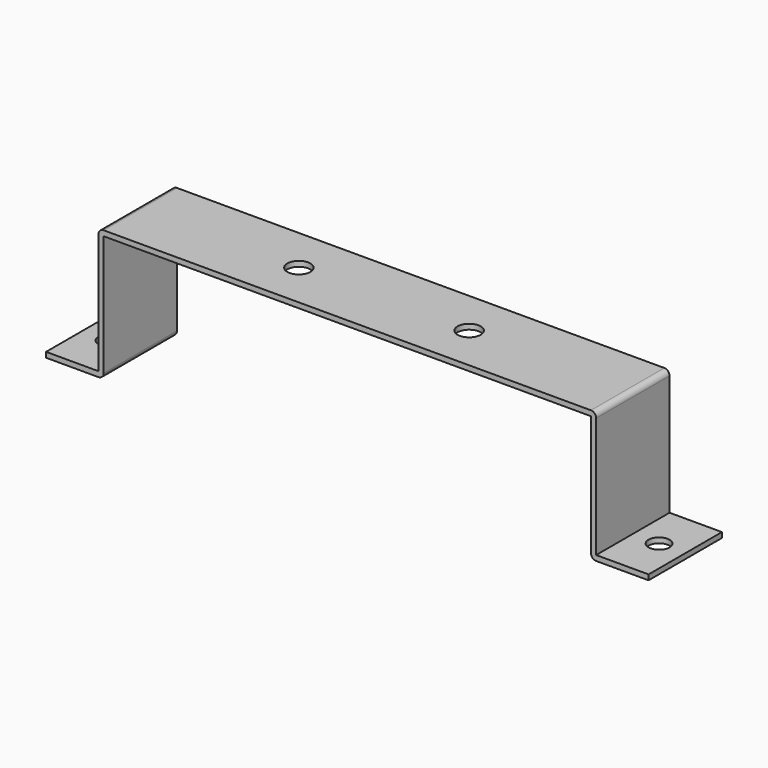
from build123d import *

# Parameters (mm, degrees)
F1_DEPTH = 17.5
F2_R     = 4
F3_DEPTH = 25
F4_R     = 4.4
F5_DEPTH = 25
F6_R     = 2


# Not quite as in the source:
# - a feature names something its author has since deleted; it is built from what else it names


with BuildPart() as f1:
    # F0 (on Front) → F1 (new body, symmetric)
    with BuildSketch(Plane.XZ):
        Polygon((95, -38), (95, 10), (-95, 10), (-95, -38), (-115, -38), (-115, -40), (-93, -40), (-93, 8), (93, 8), (93, -40), (115, -40), (115, -38), align=None)
    extrude(amount=F1_DEPTH, both=True)

    # F2 (on face) → F3 (cut)
    with BuildSketch(Plane.XY.offset(-38)):
        with Locations((-105, 0)):
            Circle(F2_R)
        with Locations((105, 0)):
            Circle(F2_R)
    extrude(amount=-F3_DEPTH, mode=Mode.SUBTRACT)

    # F4 (on face) → F5 (cut)
    with BuildSketch(Plane.XY.offset(10)):
        with Locations((-32.5, 0)):
            Circle(F4_R)
        with Locations((32.5, 0)):
            Circle(F4_R)
    extrude(amount=-F5_DEPTH, mode=Mode.SUBTRACT)

    # F6
    f6_edges = [f1.edges().sort_by_distance(p)[0] for p in [
        (95, 0, 10),
        (-95, 0, 10),
        (-93, 0, -40),
        (93, 0, -40),
    ]]
    fillet(f6_edges, radius=F6_R)


solid = f1.part
